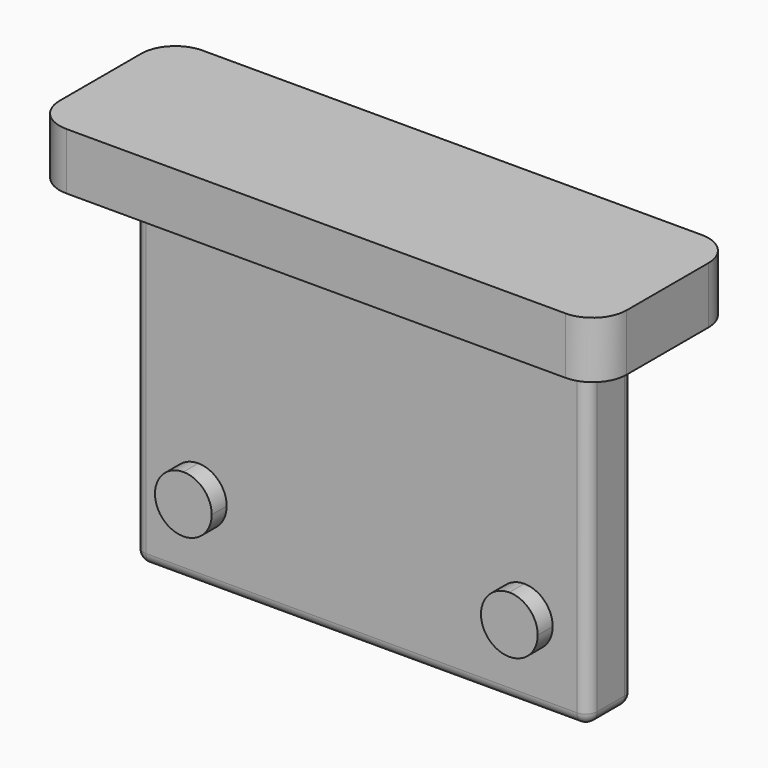
from build123d import *

# Parameters (mm, degrees)
F0_W     = 40
F0_H     = 5
F1_DEPTH = 30
F2_W     = 50
F2_H     = 15
F3_DEPTH = 5
F4_R     = 1
F5_R     = 3
F7_W     = 11.8711991236
F7_H     = 2.3502776772
F8_DEPTH = 5
F10_R    = 2.49999


# Not quite as in the source:
# - a fillet or chamfer is up to 0.001 mm smaller than in the source, because OpenCascade refuses the exact size


with BuildPart() as f1:
    # F0 (on Top) → F1 (new body)
    with BuildSketch(Plane.XY):
        Rectangle(F0_W, F0_H)
    extrude(amount=F1_DEPTH)

    # F2 (on face) → F3 (join)
    with BuildSketch(Plane.XY.offset(30)):
        Rectangle(F2_W, F2_H)
    extrude(amount=F3_DEPTH)

    # F4
    f4_edges = [f1.edges().sort_by_distance(p)[0] for p in [
        (20, 2.5, 15),
        (20, -2.5, 15),
        (-20, -2.5, 15),
        (-20, 2.5, 15),
        (0, 2.5, 0),
        (0, -2.5, 0),
        (20, 0, 0),
        (-20, 0, 0),
    ]]
    fillet(f4_edges, radius=F4_R)

    # F5
    f5_edges = [f1.edges().sort_by_distance(p)[0] for p in [
        (25, 7.5, 32.5),
        (25, -7.5, 32.5),
        (-25, 7.5, 32.5),
        (-25, -7.5, 32.5),
    ]]
    fillet(f5_edges, radius=F5_R)


with BuildPart() as f8:
    # F7 (on offset) → F8 (new body)
    with BuildSketch(Plane(origin=(0, 0, 9.5), x_dir=(1, 0, 0), z_dir=(0, 0, -1))):
        Polygon((11.8711991236, -4.8502776772), (16.8711991236, -4.8502776772), (16.8711991236, 4.1497223228), (11.8711991236, 4.1497223228), (11.8711991236, -2.5), align=None)
        with Locations((5.9355995618, -3.6751388386)):
            Rectangle(F7_W, F7_H)
    extrude(amount=F8_DEPTH)

    # F9: F8 across plane


with BuildPart() as f8_1:
    add(f8.part)
    add(f8.part.mirror(Plane.YZ))

    # F10 (radius 2.5 in the source; OpenCascade refuses exactly that, so slightly less here)
    f10_edges = [f8_1.edges().sort_by_distance(p)[0] for p in [
        (-16.871199, 0.350278, 4.5),
        (-11.871199, -0.824861, 4.5),
        (11.871199, -0.824861, 4.5),
        (16.871199, 0.350278, 4.5),
        (16.871199, 0.350278, 9.5),
        (-11.871199, -0.824861, 9.5),
        (11.871199, -0.824861, 9.5),
        (-16.871199, 0.350278, 9.5),
    ]]
    fillet(f10_edges, radius=F10_R)


solid = Compound([f1.part, f8_1.part])
